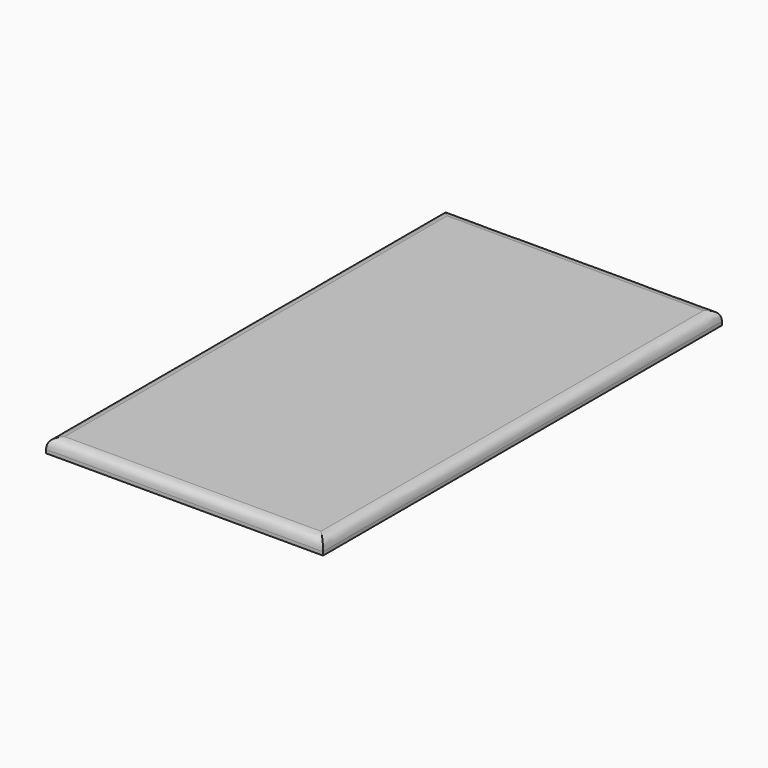
from build123d import *

# Parameters (mm, degrees)
F0_W        = 1016
F0_H        = 1828.8
F1_DEPTH    = 50.8
F2_T1_DEPTH = 1206.4995000007
F2_T3_DEPTH = 2019.2995000007


# Not quite as in the source:
# - a fillet or chamfer that OpenCascade refuses, or shapes differently, is made with other operations: its cross-section is extruded or revolved along the edge and cut away or added


with BuildPart() as f1:
    # F0 (on Top) → F1 (new body)
    with BuildSketch(Plane.XY):
        with Locations((-46.0038529815, -19.5155441761)):
            Rectangle(F0_W, F0_H)
    extrude(amount=F1_DEPTH)

    # F2: fillet of radius 38.1 on 4 edges, made by hand

    # F2_s2 → F2_t1 (cut)
    with BuildSketch(Plane.YZ.offset(-649.2536029818)):
        with BuildLine():
            add(Edge.make_bspline(
                [(-933.9156441761, 12.7001), (-933.9156441761, 50.8001), (-895.8156441761, 50.8001)],
                knots=[0, 0, 0, 1, 1, 1], degree=2, weights=[1, 1, 1]))
            Line((-895.8156441761, 50.8001), (-895.8156441761, 51.5621))
            ThreePointArc((-895.8156441761, 51.5621), (-914.8655941761, 51.562), (-933.9155441761, 51.562))
            Line((-933.9155441761, 51.562), (-934.6775441761, 50.8))
            ThreePointArc((-934.6775441761, 50.8), (-934.6775441761, 31.75005), (-934.6776441761, 12.7001))
            Line((-934.6776441761, 12.7001), (-933.9156441761, 12.7001))
        make_face()
        with BuildLine():
            add(Edge.make_bspline(
                [(894.8845558239, 12.7001), (894.8845558239, 50.8001), (856.7845558239, 50.8001)],
                knots=[0, 0, 0, 1, 1, 1], degree=2, weights=[1, 1, 1]))
            Line((856.7845558239, 50.8001), (856.7845558239, 51.5621))
            ThreePointArc((856.7845558239, 51.5621), (875.8345058239, 51.562), (894.8844558239, 51.562))
            Line((894.8844558239, 51.562), (895.6464558239, 50.8))
            ThreePointArc((895.6464558239, 50.8), (895.6464558239, 31.75005), (895.6465558239, 12.7001))
            Line((895.6465558239, 12.7001), (894.8845558239, 12.7001))
        make_face()
    extrude(amount=F2_T1_DEPTH, mode=Mode.SUBTRACT)

    # F2_s4 → F2_t3 (cut)
    with BuildSketch(Plane.XZ.offset(-990.1342058242)):
        with BuildLine():
            add(Edge.make_bspline(
                [(461.9962470185, 12.7001), (461.9962470185, 50.8001), (423.8962470185, 50.8001)],
                knots=[0, 0, 0, 1, 1, 1], degree=2, weights=[1, 1, 1]))
            Line((423.8962470185, 50.8001), (423.8962470185, 51.5621))
            ThreePointArc((423.8962470185, 51.5621), (442.9461970185, 51.562), (461.9961470185, 51.562))
            Line((461.9961470185, 51.562), (462.7581470185, 50.8))
            ThreePointArc((462.7581470185, 50.8), (462.7581470185, 31.75005), (462.7582470185, 12.7001))
            Line((462.7582470185, 12.7001), (461.9962470185, 12.7001))
        make_face()
        with BuildLine():
            add(Edge.make_bspline(
                [(-554.0039529815, 12.7001), (-554.0039529815, 50.8001), (-515.9039529815, 50.8001)],
                knots=[0, 0, 0, 1, 1, 1], degree=2, weights=[1, 1, 1]))
            Line((-515.9039529815, 50.8001), (-515.9039529815, 51.5621))
            ThreePointArc((-515.9039529815, 51.5621), (-534.9539029815, 51.562), (-554.0038529815, 51.562))
            Line((-554.0038529815, 51.562), (-554.7658529815, 50.8))
            ThreePointArc((-554.7658529815, 50.8), (-554.7658529815, 31.75005), (-554.7659529815, 12.7001))
            Line((-554.7659529815, 12.7001), (-554.0039529815, 12.7001))
        make_face()
    extrude(amount=F2_T3_DEPTH, mode=Mode.SUBTRACT)


solid = f1.part
